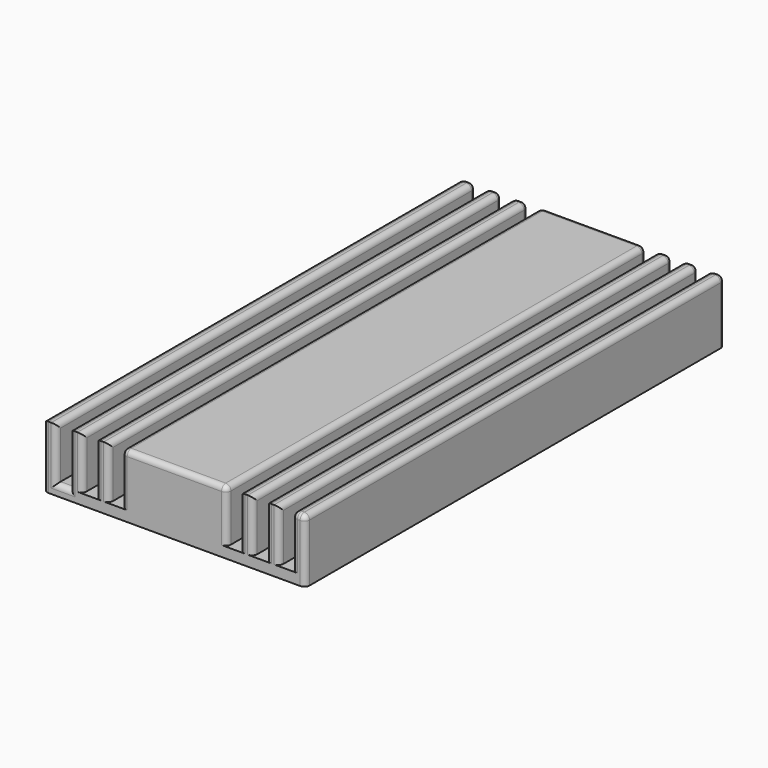
from build123d import *

# Parameters (mm, degrees)
F0_W         = 25.4
F0_H         = 50.8
F1_DEPTH     = 6.096
F2_W         = 1.27
F2_H         = 5.08
F3_DEPTH     = 50.8
F4_R         = 0.508
F5_T1_DEPTH  = 4.572
F5_T3_DEPTH  = 6.858
F5_T5_DEPTH  = 51.562
F5_T7_DEPTH  = 8.636
F5_T9_DEPTH  = 0.254
F5_T11_DEPTH = 0.254
F5_T13_DEPTH = 0.254
F5_T15_DEPTH = 0.254
F5_T17_DEPTH = 9.144
F5_T19_DEPTH = 0.254
F5_T21_DEPTH = 0.254
F5_S25_W     = 0.508
F5_S25_H     = 0.508
F5_T26_DEPTH = 0.508
F5_S31_W     = 0.508
F5_S31_H     = 0.508
F5_T32_DEPTH = 0.508
F5_T36_ANGLE = 90
F5_T38_ANGLE = 90
F5_T40_ANGLE = 90
F5_T42_ANGLE = 90
F5_T44_ANGLE = 90
F5_T46_ANGLE = 90
F5_T48_ANGLE = 90
F5_T50_ANGLE = 90
F5_T52_ANGLE = 90
F5_T54_ANGLE = 90
F5_T56_ANGLE = 90
F5_T58_ANGLE = 90
F5_T60_ANGLE = 90
F5_T62_ANGLE = 90


# Not quite as in the source:
# - a fillet or chamfer that OpenCascade refuses, or shapes differently, is made with other operations: its cross-section is extruded or revolved along the edge and cut away or added


with BuildPart() as f1:
    # F0 (on Top) → F1 (new body)
    with BuildSketch(Plane.XY):
        Rectangle(F0_W, F0_H)
    extrude(amount=F1_DEPTH)

    # F2 (on face) → F3 (cut)
    with BuildSketch(Plane.XZ.offset(25.4)):
        with Locations((-10.795, 3.556)):
            Rectangle(F2_W, F2_H)
        with Locations((-8.255, 3.556)):
            Rectangle(F2_W, F2_H)
        with Locations((-5.715, 3.556)):
            Rectangle(F2_W, F2_H)
        with Locations((5.715, 3.556)):
            Rectangle(F2_W, F2_H)
        with Locations((8.255, 3.556)):
            Rectangle(F2_W, F2_H)
        with Locations((10.795, 3.556)):
            Rectangle(F2_W, F2_H)
    extrude(amount=-F3_DEPTH, mode=Mode.SUBTRACT)

    # F4
    f4_edges = [f1.edges().sort_by_distance(p)[0] for p in [
        (-11.43, 0, 6.096),
        (-10.16, 0, 6.096),
        (-8.89, 0, 6.096),
        (-7.62, 0, 6.096),
        (-6.35, 0, 6.096),
        (-5.08, 0, 6.096),
        (5.08, 0, 6.096),
        (6.35, 0, 6.096),
        (7.62, 0, 6.096),
        (8.89, 0, 6.096),
        (10.16, 0, 6.096),
        (11.43, 0, 6.096),
        (12.7, 0, 6.096),
        (0, -25.4, 6.096),
        (-11.43, -25.4, 3.556),
        (-10.795, -25.4, 1.016),
        (-10.16, -25.4, 3.556),
        (-8.89, -25.4, 3.556),
        (-7.62, -25.4, 3.556),
        (-6.35, -25.4, 3.556),
        (-5.08, -25.4, 3.556),
        (5.08, -25.4, 3.556),
        (7.62, -25.4, 3.556),
        (6.35, -25.4, 3.556),
        (10.16, -25.4, 3.556),
        (8.89, -25.4, 3.556),
        (11.43, -25.4, 3.556),
    ]]
    fillet(f4_edges, radius=F4_R)

    # F5: fillet of radius 0.508 on 11 edges, made by hand

    # F5_s2 → F5_t1 (cut)
    with BuildSketch(Plane.XY.offset(1.016)):
        with BuildLine():
            ThreePointArc((9.398, 25.4), (9.0387897552, 25.2512102448), (8.89, 24.892))
            Line((8.89, 24.892), (8.89, 25.4))
            Line((8.89, 25.4), (9.398, 25.4))
        make_face()
        with BuildLine():
            ThreePointArc((7.112, 25.4), (7.4712102448, 25.2512102448), (7.62, 24.892))
            Line((7.62, 24.892), (7.62, 25.4))
            Line((7.62, 25.4), (7.112, 25.4))
        make_face()
        with BuildLine():
            ThreePointArc((4.572, 25.4), (4.9312102448, 25.2512102448), (5.08, 24.892))
            Line((5.08, 24.892), (5.08, 25.4))
            Line((5.08, 25.4), (4.572, 25.4))
        make_face()
        with BuildLine():
            ThreePointArc((-7.112, 25.4), (-7.4712102448, 25.2512102448), (-7.62, 24.892))
            Line((-7.62, 24.892), (-7.62, 25.4))
            Line((-7.62, 25.4), (-7.112, 25.4))
        make_face()
        with BuildLine():
            ThreePointArc((-9.398, 25.4), (-9.0387897552, 25.2512102448), (-8.89, 24.892))
            Line((-8.89, 24.892), (-8.89, 25.4))
            Line((-8.89, 25.4), (-9.398, 25.4))
        make_face()
        with BuildLine():
            ThreePointArc((-11.938, 25.4), (-11.5787897552, 25.2512102448), (-11.43, 24.892))
            Line((-11.43, 24.892), (-11.43, 25.4))
            Line((-11.43, 25.4), (-11.938, 25.4))
        make_face()
        with BuildLine():
            ThreePointArc((11.938, 25.4), (11.5787897552, 25.2512102448), (11.43, 24.892))
            Line((11.43, 24.892), (11.43, 25.4))
            Line((11.43, 25.4), (11.938, 25.4))
        make_face()
        with BuildLine():
            ThreePointArc((-9.652, 25.4), (-10.0112102448, 25.2512102448), (-10.16, 24.892))
            Line((-10.16, 24.892), (-10.16, 25.4))
            Line((-10.16, 25.4), (-9.652, 25.4))
        make_face()
        with BuildLine():
            ThreePointArc((-6.858, 25.4), (-6.4987897552, 25.2512102448), (-6.35, 24.892))
            Line((-6.35, 24.892), (-6.35, 25.4))
            Line((-6.35, 25.4), (-6.858, 25.4))
        make_face()
        with BuildLine():
            ThreePointArc((-4.572, 25.4), (-4.9312102448, 25.2512102448), (-5.08, 24.892))
            Line((-5.08, 24.892), (-5.08, 25.4))
            Line((-5.08, 25.4), (-4.572, 25.4))
        make_face()
        with BuildLine():
            ThreePointArc((6.858, 25.4), (6.4987897552, 25.2512102448), (6.35, 24.892))
            Line((6.35, 24.892), (6.35, 25.4))
            Line((6.35, 25.4), (6.858, 25.4))
        make_face()
        with BuildLine():
            ThreePointArc((9.652, 25.4), (10.0112102448, 25.2512102448), (10.16, 24.892))
            Line((10.16, 24.892), (10.16, 25.4))
            Line((10.16, 25.4), (9.652, 25.4))
        make_face()
    extrude(amount=F5_T1_DEPTH, mode=Mode.SUBTRACT)

    # F5_s4 → F5_t3 (cut)
    with BuildSketch(Plane.XY.offset(-1.27)):
        with BuildLine():
            ThreePointArc((-12.192, 25.4), (-12.5512102448, 25.2512102448), (-12.7, 24.892))
            Line((-12.7, 24.892), (-12.7, 25.4))
            Line((-12.7, 25.4), (-12.192, 25.4))
        make_face()
        with BuildLine():
            ThreePointArc((12.7, -24.892), (12.5512102448, -25.2512102448), (12.192, -25.4))
            Line((12.192, -25.4), (12.7, -25.4))
            Line((12.7, -25.4), (12.7, -24.892))
        make_face()
        with BuildLine():
            ThreePointArc((12.7, 24.892), (12.5512102448, 25.2512102448), (12.192, 25.4))
            Line((12.192, 25.4), (12.7, 25.4))
            Line((12.7, 25.4), (12.7, 24.892))
        make_face()
    extrude(amount=F5_T3_DEPTH, mode=Mode.SUBTRACT)

    # F5_s6 → F5_t5 (cut)
    with BuildSketch(Plane.XZ.offset(-24.892)):
        with BuildLine():
            ThreePointArc((-12.7, 5.588), (-12.5512102448, 5.9472102448), (-12.192, 6.096))
            Line((-12.192, 6.096), (-12.7, 6.096))
            Line((-12.7, 6.096), (-12.7, 5.588))
        make_face()
    extrude(amount=F5_T5_DEPTH, mode=Mode.SUBTRACT)

    # F5_s8 → F5_t7 (cut)
    with BuildSketch(Plane.XY.offset(-1.27)):
        with BuildLine():
            ThreePointArc((-12.192, -25.4), (-12.5512102448, -25.2512102448), (-12.7, -24.892))
            Line((-12.7, -24.892), (-12.7, -25.4))
            Line((-12.7, -25.4), (-12.192, -25.4))
        make_face()
    extrude(amount=F5_T7_DEPTH, mode=Mode.SUBTRACT)

    # F5_s10 → F5_t9 (cut)
    with BuildSketch(Plane.YZ.offset(11.938)):
        with BuildLine():
            ThreePointArc((-25.4, 5.588), (-25.2512102448, 5.9472102448), (-24.892, 6.096))
            Line((-24.892, 6.096), (-25.4, 6.096))
            Line((-25.4, 6.096), (-25.4, 5.588))
        make_face()
        with BuildLine():
            ThreePointArc((25.4, 5.588), (25.2512102448, 5.9472102448), (24.892, 6.096))
            Line((24.892, 6.096), (25.4, 6.096))
            Line((25.4, 6.096), (25.4, 5.588))
        make_face()
    extrude(amount=F5_T9_DEPTH, mode=Mode.SUBTRACT)

    # F5_s12 → F5_t11 (cut)
    with BuildSketch(Plane.YZ.offset(-12.192)):
        with BuildLine():
            ThreePointArc((25.4, 5.588), (25.2512102448, 5.9472102448), (24.892, 6.096))
            Line((24.892, 6.096), (25.4, 6.096))
            Line((25.4, 6.096), (25.4, 5.588))
        make_face()
    extrude(amount=F5_T11_DEPTH, mode=Mode.SUBTRACT)

    # F5_s14 → F5_t13 (cut)
    with BuildSketch(Plane.YZ.offset(-9.652)):
        with BuildLine():
            ThreePointArc((25.4, 5.588), (25.2512102448, 5.9472102448), (24.892, 6.096))
            Line((24.892, 6.096), (25.4, 6.096))
            Line((25.4, 6.096), (25.4, 5.588))
        make_face()
    extrude(amount=F5_T13_DEPTH, mode=Mode.SUBTRACT)

    # F5_s16 → F5_t15 (cut)
    with BuildSketch(Plane.YZ.offset(-7.112)):
        with BuildLine():
            ThreePointArc((25.4, 5.588), (25.2512102448, 5.9472102448), (24.892, 6.096))
            Line((24.892, 6.096), (25.4, 6.096))
            Line((25.4, 6.096), (25.4, 5.588))
        make_face()
    extrude(amount=F5_T15_DEPTH, mode=Mode.SUBTRACT)

    # F5_s18 → F5_t17 (cut)
    with BuildSketch(Plane.YZ.offset(-4.572)):
        with BuildLine():
            ThreePointArc((25.4, 5.588), (25.2512102448, 5.9472102448), (24.892, 6.096))
            Line((24.892, 6.096), (25.4, 6.096))
            Line((25.4, 6.096), (25.4, 5.588))
        make_face()
    extrude(amount=F5_T17_DEPTH, mode=Mode.SUBTRACT)

    # F5_s20 → F5_t19 (cut)
    with BuildSketch(Plane.YZ.offset(6.858)):
        with BuildLine():
            ThreePointArc((25.4, 5.588), (25.2512102448, 5.9472102448), (24.892, 6.096))
            Line((24.892, 6.096), (25.4, 6.096))
            Line((25.4, 6.096), (25.4, 5.588))
        make_face()
    extrude(amount=F5_T19_DEPTH, mode=Mode.SUBTRACT)

    # F5_s22 → F5_t21 (cut)
    with BuildSketch(Plane.YZ.offset(9.398)):
        with BuildLine():
            ThreePointArc((25.4, 5.588), (25.2512102448, 5.9472102448), (24.892, 6.096))
            Line((24.892, 6.096), (25.4, 6.096))
            Line((25.4, 6.096), (25.4, 5.588))
        make_face()
    extrude(amount=F5_T21_DEPTH, mode=Mode.SUBTRACT)


with BuildPart() as f5_tool24:
    # F5_s25 → F5_t26 (new body)
    with BuildSketch(Plane.XZ.offset(24.892)):
        with Locations((11.684, 5.842)):
            Rectangle(F5_S25_W, F5_S25_H)
    extrude(amount=F5_T26_DEPTH)

    # F5_s27 → F5_t28 (revolve, cut)
    with BuildSketch(Plane(origin=(11.938, -24.892, 5.588), x_dir=(0.7071067812, 0, -0.7071067812), z_dir=(-0.7071067812, 0, -0.7071067812))):
        with BuildLine():
            ThreePointArc((0, -0.508), (0.508, 0), (0, 0.508))
            Line((0, 0.508), (0, -0.508))
        make_face()
    revolve(axis=Axis((11.938, -24.892, 5.588), (0, -1, 0)), mode=Mode.SUBTRACT)


with BuildPart() as f1_1:
    add(f1.part)

    # F5_t23: cut F5_tool24
    add(f5_tool24.part, mode=Mode.SUBTRACT)


with BuildPart() as f5_tool30:
    # F5_s31 → F5_t32 (new body)
    with BuildSketch(Plane.XY.offset(5.588)):
        with Locations((-12.446, 25.146)):
            Rectangle(F5_S31_W, F5_S31_H)
    extrude(amount=F5_T32_DEPTH)

    # F5_s33 → F5_t34 (revolve, cut)
    with BuildSketch(Plane(origin=(-12.192, 24.892, 5.588), x_dir=(0.7071067812, -0.7071067812, 0), z_dir=(-0.7071067812, -0.7071067812, 0))):
        with BuildLine():
            ThreePointArc((0, -0.508), (0.508, 0), (0, 0.508))
            Line((0, 0.508), (0, -0.508))
        make_face()
    revolve(axis=Axis((-12.192, 24.892, 5.588), (0, 0, 1)), mode=Mode.SUBTRACT)


with BuildPart() as f1_2:
    add(f1_1.part)

    # F5_t29: cut F5_tool30
    add(f5_tool30.part, mode=Mode.SUBTRACT)

    # F5_s35 → F5_t36 (revolve, cut)
    with BuildSketch(Plane.XY.offset(5.588)):
        with BuildLine():
            ThreePointArc((12.192, -25.4), (12.5512102448, -25.2512102448), (12.7, -24.892))
            Line((12.7, -24.892), (12.7, -25.4))
            Line((12.7, -25.4), (12.192, -25.4))
        make_face()
    revolve(axis=Axis((12.192, -25.4, 5.588), (0, -1, 0)), revolution_arc=F5_T36_ANGLE, mode=Mode.SUBTRACT)

    # F5_s37 → F5_t38 (revolve, cut)
    with BuildSketch(Plane.YZ.offset(11.938)):
        with BuildLine():
            ThreePointArc((25.4, 5.588), (25.2512102448, 5.9472102448), (24.892, 6.096))
            Line((24.892, 6.096), (25.4, 6.096))
            Line((25.4, 6.096), (25.4, 5.588))
        make_face()
    revolve(axis=Axis((11.938, 25.4, 5.588), (0, -1, 0)), revolution_arc=F5_T38_ANGLE, mode=Mode.SUBTRACT)

    # F5_s39 → F5_t40 (revolve, cut)
    with BuildSketch(Plane.XY.offset(5.588)):
        with BuildLine():
            ThreePointArc((12.7, 24.892), (12.5512102448, 25.2512102448), (12.192, 25.4))
            Line((12.192, 25.4), (12.7, 25.4))
            Line((12.7, 25.4), (12.7, 24.892))
        make_face()
    revolve(axis=Axis((12.192, 25.4, 5.588), (0, -1, 0)), revolution_arc=F5_T40_ANGLE, mode=Mode.SUBTRACT)

    # F5_s41 → F5_t42 (revolve, cut)
    with BuildSketch(Plane.XY.offset(5.588)):
        with BuildLine():
            ThreePointArc((-11.938, 25.4), (-11.5787897552, 25.2512102448), (-11.43, 24.892))
            Line((-11.43, 24.892), (-11.43, 25.4))
            Line((-11.43, 25.4), (-11.938, 25.4))
        make_face()
    revolve(axis=Axis((-11.938, 25.4, 5.588), (0, -1, 0)), revolution_arc=F5_T42_ANGLE, mode=Mode.SUBTRACT)

    # F5_s43 → F5_t44 (revolve, cut)
    with BuildSketch(Plane.XY.offset(5.588)):
        with BuildLine():
            ThreePointArc((-9.398, 25.4), (-9.0387897552, 25.2512102448), (-8.89, 24.892))
            Line((-8.89, 24.892), (-8.89, 25.4))
            Line((-8.89, 25.4), (-9.398, 25.4))
        make_face()
    revolve(axis=Axis((-9.398, 25.4, 5.588), (0, -1, 0)), revolution_arc=F5_T44_ANGLE, mode=Mode.SUBTRACT)

    # F5_s45 → F5_t46 (revolve, cut)
    with BuildSketch(Plane.YZ.offset(-9.652)):
        with BuildLine():
            ThreePointArc((25.4, 5.588), (25.2512102448, 5.9472102448), (24.892, 6.096))
            Line((24.892, 6.096), (25.4, 6.096))
            Line((25.4, 6.096), (25.4, 5.588))
        make_face()
    revolve(axis=Axis((-9.652, 25.4, 5.588), (0, -1, 0)), revolution_arc=F5_T46_ANGLE, mode=Mode.SUBTRACT)

    # F5_s47 → F5_t48 (revolve, cut)
    with BuildSketch(Plane.YZ.offset(-7.112)):
        with BuildLine():
            ThreePointArc((25.4, 5.588), (25.2512102448, 5.9472102448), (24.892, 6.096))
            Line((24.892, 6.096), (25.4, 6.096))
            Line((25.4, 6.096), (25.4, 5.588))
        make_face()
    revolve(axis=Axis((-7.112, 25.4, 5.588), (0, -1, 0)), revolution_arc=F5_T48_ANGLE, mode=Mode.SUBTRACT)

    # F5_s49 → F5_t50 (revolve, cut)
    with BuildSketch(Plane.XY.offset(5.588)):
        with BuildLine():
            ThreePointArc((-6.858, 25.4), (-6.4987897552, 25.2512102448), (-6.35, 24.892))
            Line((-6.35, 24.892), (-6.35, 25.4))
            Line((-6.35, 25.4), (-6.858, 25.4))
        make_face()
    revolve(axis=Axis((-6.858, 25.4, 5.588), (0, -1, 0)), revolution_arc=F5_T50_ANGLE, mode=Mode.SUBTRACT)

    # F5_s51 → F5_t52 (revolve, cut)
    with BuildSketch(Plane.XY.offset(5.588)):
        with BuildLine():
            ThreePointArc((4.572, 25.4), (4.9312102448, 25.2512102448), (5.08, 24.892))
            Line((5.08, 24.892), (5.08, 25.4))
            Line((5.08, 25.4), (4.572, 25.4))
        make_face()
    revolve(axis=Axis((4.572, 25.4, 5.588), (0, -1, 0)), revolution_arc=F5_T52_ANGLE, mode=Mode.SUBTRACT)

    # F5_s53 → F5_t54 (revolve, cut)
    with BuildSketch(Plane.YZ.offset(-4.572)):
        with BuildLine():
            ThreePointArc((25.4, 5.588), (25.2512102448, 5.9472102448), (24.892, 6.096))
            Line((24.892, 6.096), (25.4, 6.096))
            Line((25.4, 6.096), (25.4, 5.588))
        make_face()
    revolve(axis=Axis((-4.572, 25.4, 5.588), (0, -1, 0)), revolution_arc=F5_T54_ANGLE, mode=Mode.SUBTRACT)

    # F5_s55 → F5_t56 (revolve, cut)
    with BuildSketch(Plane.XY.offset(5.588)):
        with BuildLine():
            ThreePointArc((7.112, 25.4), (7.4712102448, 25.2512102448), (7.62, 24.892))
            Line((7.62, 24.892), (7.62, 25.4))
            Line((7.62, 25.4), (7.112, 25.4))
        make_face()
    revolve(axis=Axis((7.112, 25.4, 5.588), (0, -1, 0)), revolution_arc=F5_T56_ANGLE, mode=Mode.SUBTRACT)

    # F5_s57 → F5_t58 (revolve, cut)
    with BuildSketch(Plane.YZ.offset(6.858)):
        with BuildLine():
            ThreePointArc((25.4, 5.588), (25.2512102448, 5.9472102448), (24.892, 6.096))
            Line((24.892, 6.096), (25.4, 6.096))
            Line((25.4, 6.096), (25.4, 5.588))
        make_face()
    revolve(axis=Axis((6.858, 25.4, 5.588), (0, -1, 0)), revolution_arc=F5_T58_ANGLE, mode=Mode.SUBTRACT)

    # F5_s59 → F5_t60 (revolve, cut)
    with BuildSketch(Plane.YZ.offset(9.398)):
        with BuildLine():
            ThreePointArc((25.4, 5.588), (25.2512102448, 5.9472102448), (24.892, 6.096))
            Line((24.892, 6.096), (25.4, 6.096))
            Line((25.4, 6.096), (25.4, 5.588))
        make_face()
    revolve(axis=Axis((9.398, 25.4, 5.588), (0, -1, 0)), revolution_arc=F5_T60_ANGLE, mode=Mode.SUBTRACT)

    # F5_s61 → F5_t62 (revolve, cut)
    with BuildSketch(Plane.XY.offset(5.588)):
        with BuildLine():
            ThreePointArc((9.652, 25.4), (10.0112102448, 25.2512102448), (10.16, 24.892))
            Line((10.16, 24.892), (10.16, 25.4))
            Line((10.16, 25.4), (9.652, 25.4))
        make_face()
    revolve(axis=Axis((9.652, 25.4, 5.588), (0, -1, 0)), revolution_arc=F5_T62_ANGLE, mode=Mode.SUBTRACT)


solid = f1_2.part
